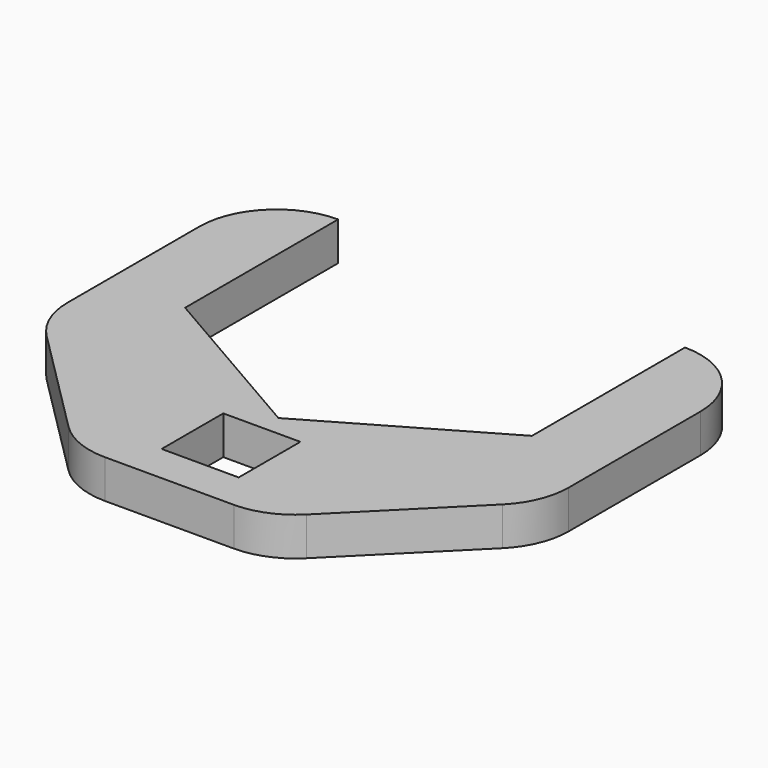
from build123d import *

# Parameters (mm, degrees)
F1_DEPTH = 5
F2_SIZE  = 20
F3_R     = 9.99999


# Not quite as in the source:
# - a fillet or chamfer is up to 0.001 mm smaller than in the source, because OpenCascade refuses the exact size
# - a feature names something its author has since deleted; it is built from what else it names


with BuildPart() as f1:
    # F0 (on Top) → F1 (new body)
    with BuildSketch(Plane.XY):
        Polygon((0, -28.6713610368), (0, -25.9807621135), (-11.250000041, -19.4855715615), (-22.5, -12.9903810568), (-22.5, 0), (-22.5, 11.8356805184), (-32.5, 11.8356805184), (-32.5, -43.6713610368), (0, -43.6713610368), (0, -38.6713610368), (-5, -38.6713610368), (-5, -28.6713610368), align=None)
        Polygon((11.2499998166, -19.485571691), (0, -25.9807621135), (0, -28.6713610368), (5, -28.6713610368), (5, -38.6713610368), (0, -38.6713610368), (0, -43.6713610368), (32.5, -43.6713610368), (32.5, 11.8356805184), (22.5, 11.8356805184), (22.5, 0), (22.5, -12.9903810568), align=None)
    extrude(amount=F1_DEPTH)

    # F2
    f2_edges = [f1.edges().sort_by_distance(p)[0] for p in [
        (-32.5, -43.671361, 2.5),
        (32.5, -43.671361, 2.5),
    ]]
    chamfer(f2_edges, length=F2_SIZE)

    # F3 (radius 10 in the source; OpenCascade refuses exactly that, so slightly less here)
    f3_edges = [f1.edges().sort_by_distance(p)[0] for p in [
        (-32.5, 11.835681, 2.5),
        (32.5, -23.671361, 2.5),
        (32.5, 11.835681, 2.5),
        (12.5, -43.671361, 2.5),
        (-12.5, -43.671361, 2.5),
        (-32.5, -23.671361, 2.5),
    ]]
    fillet(f3_edges, radius=F3_R)


solid = f1.part
